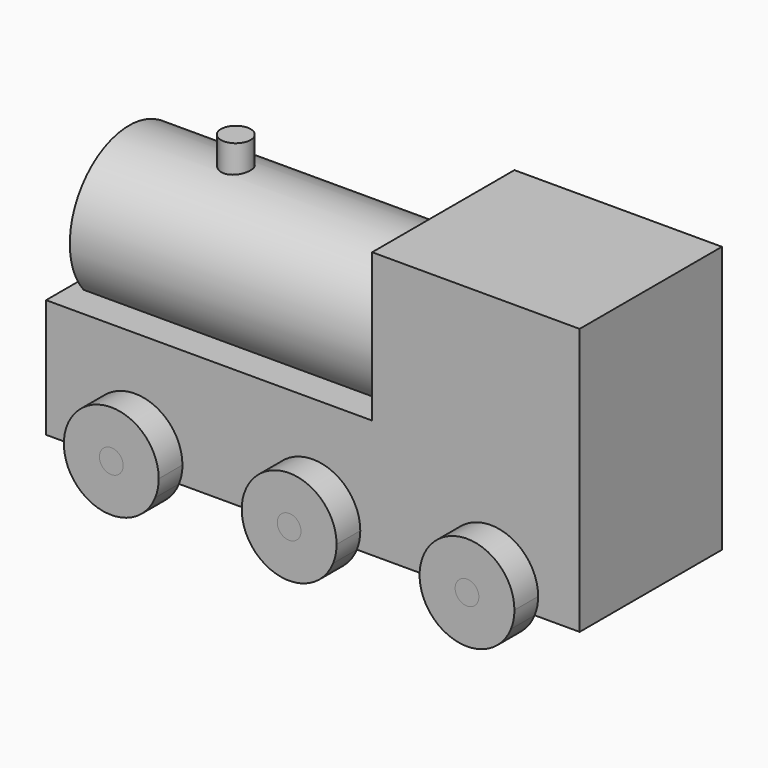
from build123d import *

# Parameters (mm, degrees)
F0_W      = 90
F0_H      = 30
F1_DEPTH  = 20
F2_W      = 35
F2_H      = 30
F3_DEPTH  = 25
F5_DEPTH  = 53
F6_R      = 2.5
F7_DEPTH  = 69.3
F8_R      = 2.5
F9_DEPTH  = 25
F11_DEPTH = 5
F14_R     = 2
F15_DEPTH = 56.1
F16_R     = 2
F17_DEPTH = 40


with BuildPart() as f1:
    # F0 (on Top) → F1 (new body)
    with BuildSketch(Plane.XY):
        with Locations((-45, -15)):
            Rectangle(F0_W, F0_H)
    extrude(amount=F1_DEPTH)

    # F2 (on face) → F3 (join)
    with BuildSketch(Plane.XY.offset(20)):
        with Locations((-17.5, -15)):
            Rectangle(F2_W, F2_H)
    extrude(amount=F3_DEPTH)

    # F8 (on face) → F9 (join)
    with BuildSketch(Plane.XY.offset(20)):
        with Locations((-70, -15)):
            Circle(F8_R)
    extrude(amount=F9_DEPTH)


with BuildPart() as f5:
    # F4 (on face) → F5 (new body)
    with BuildSketch(Plane(origin=(-35, 0, 0), x_dir=(0, -1, 0), z_dir=(-1, 0, 0))):
        with BuildLine():
            Line((5.3953136439, 20), (24.6046863561, 20))
            ThreePointArc((24.6046863561, 20), (15, 40.5), (5.3953136439, 20))
        make_face()
    extrude(amount=F5_DEPTH)

    # F6 (on face) → F7 (cut)
    with BuildSketch(Plane.XY.offset(45)):
        with Locations((-70, -15)):
            Circle(F6_R)
    extrude(amount=-F7_DEPTH, mode=Mode.SUBTRACT)


with BuildPart() as f11:
    # F10 (on face) → F11 (new body)
    with BuildSketch(Plane.XZ.offset(30)):
        with BuildLine():
            Line((-67.5838015129, 0), (-82.4161984871, 0))
            ThreePointArc((-82.4161984871, 0), (-75, -5), (-67.5838015129, 0))
        make_face()
        with BuildLine():
            ThreePointArc((-67.5838015129, 0), (-67.14730658, 1.4718619003), (-67, 3))
            ThreePointArc((-67, 3), (-76.5281380997, 10.85269342), (-82.4161984871, 0))
            Line((-82.4161984871, 0), (-67.5838015129, 0))
        make_face()
    extrude(amount=F11_DEPTH)


with BuildPart() as f11b:
    # F10 (on face) → F11, piece 2 (new body)
    with BuildSketch(Plane.XZ.offset(30)):
        with BuildLine():
            ThreePointArc((-37, 3), (-46.5281380997, 10.85269342), (-52.4161984871, 0))
            Line((-52.4161984871, 0), (-37.5838015129, 0))
            ThreePointArc((-37.5838015129, 0), (-37.14730658, 1.4718619003), (-37, 3))
        make_face()
        with BuildLine():
            Line((-37.5838015129, 0), (-52.4161984871, 0))
            ThreePointArc((-52.4161984871, 0), (-45, -5), (-37.5838015129, 0))
        make_face()
    extrude(amount=F11_DEPTH)


with BuildPart() as f11c:
    # F10 (on face) → F11, piece 3 (new body)
    with BuildSketch(Plane.XZ.offset(30)):
        with BuildLine():
            ThreePointArc((-7, 3), (-16.5281380997, 10.85269342), (-22.4161984871, 0))
            Line((-22.4161984871, 0), (-7.5838015129, 0))
            ThreePointArc((-7.5838015129, 0), (-7.14730658, 1.4718619003), (-7, 3))
        make_face()
        with BuildLine():
            Line((-7.5838015129, 0), (-22.4161984871, 0))
            ThreePointArc((-22.4161984871, 0), (-15, -5), (-7.5838015129, 0))
        make_face()
    extrude(amount=F11_DEPTH)


with BuildPart() as f13_1:
    # F13: instance of F11
    add(f11.part.mirror(Plane.XZ.offset(15)))


with BuildPart() as f13_2:
    # F13: instance of F11b
    add(f11b.part.mirror(Plane.XZ.offset(15)))


with BuildPart() as f13_3:
    # F13: instance of F11c
    add(f11c.part.mirror(Plane.XZ.offset(15)))


with BuildPart() as f15_tool:
    # F14 (on face) → F15 (new body)
    with BuildSketch(Plane.XZ.offset(35)):
        with Locations((-45, 3)):
            Circle(F14_R)
        with Locations((-15, 3)):
            Circle(F14_R)
        with Locations((-75, 3)):
            Circle(F14_R)
    extrude(amount=-F15_DEPTH)


with BuildPart() as f1_1:
    add(f1.part)

    # F15: cut by f15_tool
    add(f15_tool.part, mode=Mode.SUBTRACT)


with BuildPart() as f11_1:
    add(f11.part)

    # F15: cut by f15_tool
    add(f15_tool.part, mode=Mode.SUBTRACT)


with BuildPart() as f11b_1:
    add(f11b.part)

    # F15: cut by f15_tool
    add(f15_tool.part, mode=Mode.SUBTRACT)


with BuildPart() as f11c_1:
    add(f11c.part)

    # F15: cut by f15_tool
    add(f15_tool.part, mode=Mode.SUBTRACT)


with BuildPart() as f13_1_1:
    add(f13_1.part)

    # F15: cut by f15_tool
    add(f15_tool.part, mode=Mode.SUBTRACT)


with BuildPart() as f13_2_1:
    add(f13_2.part)

    # F15: cut by f15_tool
    add(f15_tool.part, mode=Mode.SUBTRACT)


with BuildPart() as f13_3_1:
    add(f13_3.part)

    # F15: cut by f15_tool
    add(f15_tool.part, mode=Mode.SUBTRACT)


with BuildPart() as f17:
    # F16 (on face) → F17 (new body, through all)
    with BuildSketch(Plane.XZ.offset(35)):
        with Locations((-75, 3)):
            Circle(F16_R)
    extrude(amount=-F17_DEPTH)


with BuildPart() as f17b:
    # F16 (on face) → F17, piece 2 (new body, through all)
    with BuildSketch(Plane.XZ.offset(35)):
        with Locations((-45, 3)):
            Circle(F16_R)
    extrude(amount=-F17_DEPTH)


with BuildPart() as f17c:
    # F16 (on face) → F17, piece 3 (new body, through all)
    with BuildSketch(Plane.XZ.offset(35)):
        with Locations((-15, 3)):
            Circle(F16_R)
    extrude(amount=-F17_DEPTH)


solid = Compound([f5.part, f1_1.part, f11_1.part, f11b_1.part, f11c_1.part, f13_1_1.part, f13_2_1.part, f13_3_1.part, f17.part, f17b.part, f17c.part])
